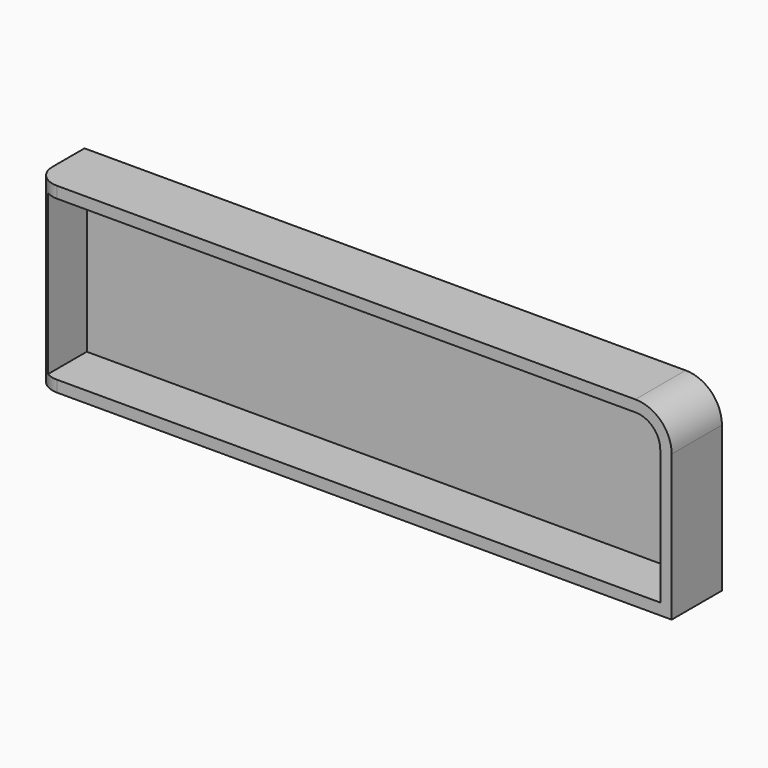
from build123d import *

# Parameters (mm, degrees)
F0_W        = 140
F0_H        = 40
F1_DEPTH    = 13.8
F2_R        = 7.9669047558
F3_T        = -2.5
F4_T1_DEPTH = 65


# Not quite as in the source:
# - a fillet or chamfer that OpenCascade refuses, or shapes differently, is made with other operations: its cross-section is extruded or revolved along the edge and cut away or added


with BuildPart() as f1:
    # F0 (on Front) → F1 (new body)
    with BuildSketch(Plane.XZ):
        with Locations((-0.0846795738, 4.6162967879)):
            Rectangle(F0_W, F0_H)
    extrude(amount=F1_DEPTH)

    # F2
    f2_edges = [f1.edges().sort_by_distance(p)[0] for p in [
        (69.91532, -6.9, 24.616297),
    ]]
    fillet(f2_edges, radius=F2_R)

    # F3
    f3_openings = [f1.faces().sort_by_distance(p)[0] for p in [
        (-0.25102, -13.8, 4.57187),
    ]]
    offset(amount=F3_T, openings=f3_openings)

    # F4: fillet of radius 5 on 1 edges, made by hand

    # F4_s2 → F4_t1 (cut)
    with BuildSketch(Plane.XY.offset(-27.8837032121)):
        with BuildLine():
            ThreePointArc((-70.0846795738, -8.8), (-68.6202134797, -12.3355339059), (-65.0846795738, -13.8))
            Line((-65.0846795738, -13.8), (-70.0846795738, -13.8))
            Line((-70.0846795738, -13.8), (-70.0846795738, -8.8))
        make_face()
    extrude(amount=F4_T1_DEPTH, mode=Mode.SUBTRACT)


solid = f1.part
